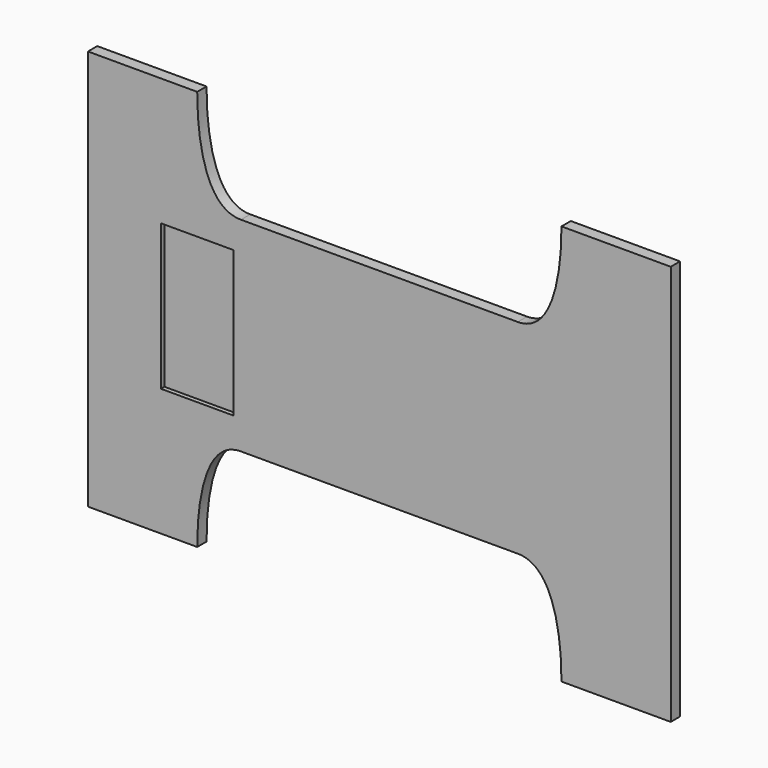
from build123d import *

# Parameters (mm, degrees)
F0_W     = 100
F0_H     = 200
F1_DEPTH = 16
F2_DEPTH = 10


# Not quite as in the source:
# - a feature names something its author has since deleted; it is built from what else it names


with BuildPart() as f1:
    # F0 (on Front) → F1 (new body)
    with BuildSketch(Plane.XZ):
        Polygon((-250, 275), (-400, 275), (-400, -275), (-250, -275), (-250, -140), (-190, -140), (190, -140), (250, -140), (250, -275), (400, -275), (400, 275), (250, 275), (250, 140), (190, 140), (-190, 140), (-250, 140), align=None)
        with Locations((-250, 0)):
            Rectangle(F0_W, F0_H, mode=Mode.SUBTRACT)
        with BuildLine():
            add(Edge.make_bspline(
                [(-250, 275), (-250, 256.6260014103), (-250, 140), (-190, 140)],
                knots=[0, 0, 0, 0, 147.7328670269, 147.7328670269, 147.7328670269, 147.7328670269], degree=3))
            Line((-250, 275), (-250, 140))
            Line((-250, 140), (-190, 140))
        make_face()
        with BuildLine():
            Line((250, 140), (250, 275))
            add(Edge.make_bspline(
                [(250, 275), (250, 256.6260014103), (250, 140), (190, 140)],
                knots=[0, 0, 0, 0, 147.7328670269, 147.7328670269, 147.7328670269, 147.7328670269], degree=3))
            Line((190, 140), (250, 140))
        make_face()
        with BuildLine():
            Line((-250, -140), (-250, -275))
            add(Edge.make_bspline(
                [(-250, -275), (-250, -256.6260014103), (-250, -140), (-190, -140)],
                knots=[0, 0, 0, 0, 147.7328670269, 147.7328670269, 147.7328670269, 147.7328670269], degree=3))
            Line((-190, -140), (-250, -140))
        make_face()
        with BuildLine():
            add(Edge.make_bspline(
                [(250, -275), (250, -256.6260014103), (250, -140), (190, -140)],
                knots=[0, 0, 0, 0, 147.7328670269, 147.7328670269, 147.7328670269, 147.7328670269], degree=3))
            Line((250, -275), (250, -140))
            Line((250, -140), (190, -140))
        make_face()
    extrude(amount=F1_DEPTH)


with BuildPart() as f2:
    # F0 (on Front) → F2 (new body)
    with BuildSketch(Plane.XZ):
        with Locations((-250, 0)):
            Rectangle(F0_W, F0_H)
    extrude(amount=F2_DEPTH)


solid = Compound([f1.part, f2.part])
